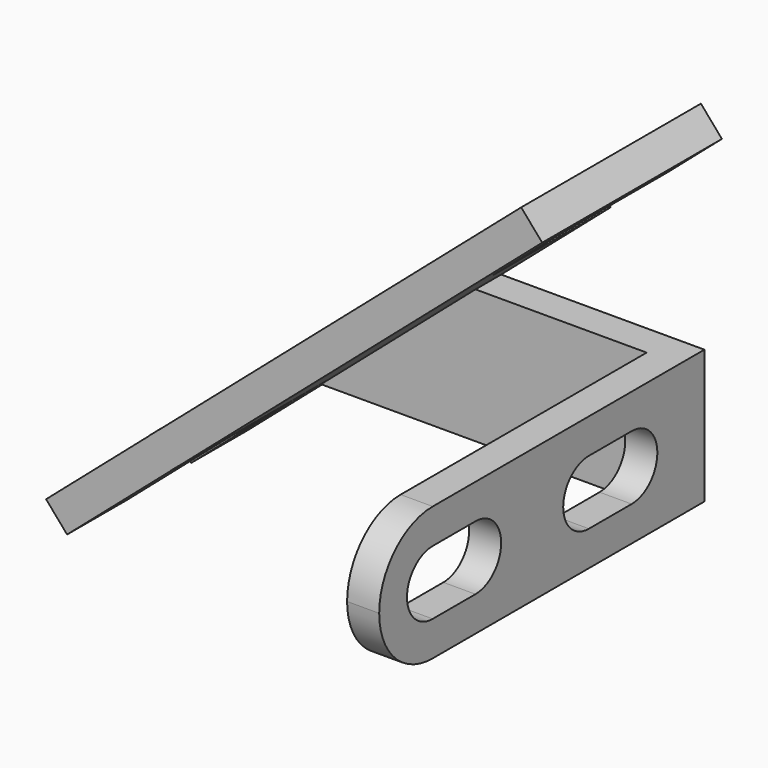
from build123d import *

# Parameters (mm, degrees)
F0_W      = 1612.9
F0_H      = 12.7
F0_H_2    = 609.6
F1_DEPTH  = 152.4
F2_W      = 254
F2_H      = 304.8
F3_DEPTH  = 152.4
F4_W      = 317.5
F4_H      = 635
F5_DEPTH  = 152.4
F6_R      = 317.49999
F8_DEPTH  = 152.4
F9_W      = 965.2
F9_H      = 635
F10_DEPTH = 152.4
F12_DEPTH = 152.4
F14_W     = 647.7
F14_H     = 1066.8
F15_DEPTH = 152.4
F16_W     = 2336.8
F16_H     = 1066.8
F17_DEPTH = 152.4
F19_DEPTH = 1066.8
F22_DEPTH = 1066.8
F23_W     = 635
F23_H     = 381
F24_DEPTH = 152.4
F25_W     = 355.6
F25_H     = 711.2
F26_DEPTH = 152.4


# Not quite as in the source:
# - a fillet or chamfer is up to 0.001 mm smaller than in the source, because OpenCascade refuses the exact size
# - a feature names something its author has since deleted; it is built from what else it names


with BuildPart() as f1:
    # F0 (on Right) → F1 (new body)
    with BuildSketch(Plane.YZ):
        with Locations((-806.45, -6.35)):
            Rectangle(F0_W, F0_H)
        with Locations((-806.45, 304.8)):
            Rectangle(F0_W, F0_H_2)
        with Locations((-806.45, 615.95)):
            Rectangle(F0_W, F0_H)
    extrude(amount=-F1_DEPTH)

    # F2 (on face) → F3 (cut)
    with BuildSketch(Plane.YZ):
        with Locations((-558.8, 304.8)):
            Rectangle(F2_W, F2_H)
        with Locations((-1485.9, 304.8)):
            Rectangle(F2_W, F2_H)
    extrude(amount=-F3_DEPTH, mode=Mode.SUBTRACT)

    # F4 (on face) → F5 (join)
    with BuildSketch(Plane.YZ):
        with Locations((-1771.65, 304.8)):
            Rectangle(F4_W, F4_H)
    extrude(amount=-F5_DEPTH)

    # F6 (radius 317.5 in the source; OpenCascade refuses exactly that, so slightly less here)
    f6_edges = [f1.edges().sort_by_distance(p)[0] for p in [
        (-76.2, -1930.4, 622.3),
        (-76.2, -1930.4, -12.7),
    ]]
    fillet(f6_edges, radius=F6_R)

    # F7 (on face) → F8 (cut)
    with BuildSketch(Plane.YZ):
        with BuildLine():
            ThreePointArc((-1485.9, 220.557730325), (-1466.9881087779, 260.8059094878), (-1460.5, 304.8))
            ThreePointArc((-1460.5, 304.8), (-1466.9881087779, 348.7940905122), (-1485.9, 389.042269675))
            ThreePointArc((-1485.9, 389.042269675), (-1511.3, 304.8), (-1485.9, 220.557730325))
        make_face()
        with BuildLine():
            ThreePointArc((-1485.9, 389.042269675), (-1466.9881087779, 348.7940905122), (-1460.5, 304.8))
            ThreePointArc((-1460.5, 304.8), (-1466.9881087779, 260.8059094878), (-1485.9, 220.557730325))
            ThreePointArc((-1485.9, 220.557730325), (-1314.9059094878, 158.8881087779), (-1206.5, 304.8))
            ThreePointArc((-1206.5, 304.8), (-1314.9059094878, 450.7118912221), (-1485.9, 389.042269675))
        make_face()
        with BuildLine():
            ThreePointArc((-1485.9, 220.557730325), (-1511.3, 304.8), (-1485.9, 389.042269675))
            ThreePointArc((-1485.9, 389.042269675), (-1765.3, 304.8), (-1485.9, 220.557730325))
        make_face()
        with BuildLine():
            ThreePointArc((-558.8, 220.557730325), (-539.8881087779, 260.8059094878), (-533.4, 304.8))
            ThreePointArc((-533.4, 304.8), (-539.8881087779, 348.7940905122), (-558.8, 389.042269675))
            ThreePointArc((-558.8, 389.042269675), (-584.2, 304.8), (-558.8, 220.557730325))
        make_face()
        with BuildLine():
            ThreePointArc((-558.8, 389.042269675), (-539.8881087779, 348.7940905122), (-533.4, 304.8))
            ThreePointArc((-533.4, 304.8), (-539.8881087779, 260.8059094878), (-558.8, 220.557730325))
            ThreePointArc((-558.8, 220.557730325), (-387.8059094878, 158.8881087779), (-279.4, 304.8))
            ThreePointArc((-279.4, 304.8), (-387.8059094878, 450.7118912221), (-558.8, 389.042269675))
        make_face()
        with BuildLine():
            ThreePointArc((-558.8, 220.557730325), (-584.2, 304.8), (-558.8, 389.042269675))
            ThreePointArc((-558.8, 389.042269675), (-838.2, 304.8), (-558.8, 220.557730325))
        make_face()
    extrude(amount=-F8_DEPTH, mode=Mode.SUBTRACT)

    # F9 (on face) → F10 (join)
    with BuildSketch(Plane(origin=(0, 0, 0), x_dir=(-1, 0, 0), z_dir=(0, 1, 0))):
        with Locations((482.6, 304.8)):
            Rectangle(F9_W, F9_H)
    extrude(amount=-F10_DEPTH)

    # F11 (on face) → F12 (join)
    with BuildSketch(Plane(origin=(0, 0, 0), x_dir=(-1, 0, 0), z_dir=(0, 1, 0))):
        Polygon((1698.4472, -12.7), (965.2, 622.3), (965.2, -12.7), align=None)
    extrude(amount=-F12_DEPTH)

    # F14 (on offset) → F15 (join)
    with BuildSketch(Plane(origin=(-721.6070671381, 0, 833.2541125657), x_dir=(0.7559344062, 0, 0.6546473658), z_dir=(-0.6546473658, 0, 0.7559344062))):
        with Locations((-1596.0768110359, -533.4)):
            Rectangle(F14_W, F14_H)
    extrude(amount=F15_DEPTH)

    # F16 (on offset) → F17 (join)
    with BuildSketch(Plane(origin=(-721.6070671381, 0, 833.2541125657), x_dir=(0.7559344062, 0, 0.6546473658), z_dir=(-0.6546473658, 0, 0.7559344062))):
        with Locations((-53.897047908, -533.4)):
            Rectangle(F16_W, F16_H)
    extrude(amount=F17_DEPTH)

    # F18 (on face) → F19 (cut)
    with BuildSketch(Plane(origin=(0, 0, 0), x_dir=(-1, 0, 0), z_dir=(0, 1, 0))):
        Polygon((16.6328412597, 1645.374205089), (-21.1158016224, 1678.0649378052), (-120.8840601663, 1562.8605342995), (-83.1354172842, 1530.1698015833), align=None)
    extrude(amount=-F19_DEPTH, mode=Mode.SUBTRACT)

    # F21 (on offset) → F22 (join)
    with BuildSketch(Plane(origin=(0, 0, 0), x_dir=(-1, 0, 0), z_dir=(0, 1, 0))):
        Polygon((1640.5618513332, 38.2444991085), (1684.7235393438, 0), (1784.4917978876, 115.2044035058), (1740.3301098771, 153.4489026143), align=None)
    extrude(amount=-F22_DEPTH)

    # F23 (on face) → F24 (cut)
    with BuildSketch(Plane(origin=(-821.375325682, 0, 948.4585160715), x_dir=(0.7559344062, 0, 0.6546473658), z_dir=(-0.6546473658, 0, 0.7559344062))):
        with Locations((-1602.4268110359, -520.7)):
            Rectangle(F23_W, F23_H)
    extrude(amount=-F24_DEPTH, mode=Mode.SUBTRACT)

    # F25 (on face) → F26 (cut)
    with BuildSketch(Plane(origin=(-821.375325682, 0, 948.4585160715), x_dir=(0.7559344062, 0, 0.6546473658), z_dir=(-0.6546473658, 0, 0.7559344062))):
        with Locations((543.866552092, -355.6)):
            Rectangle(F25_W, F25_H)
    extrude(amount=-F26_DEPTH, mode=Mode.SUBTRACT)


solid = f1.part
